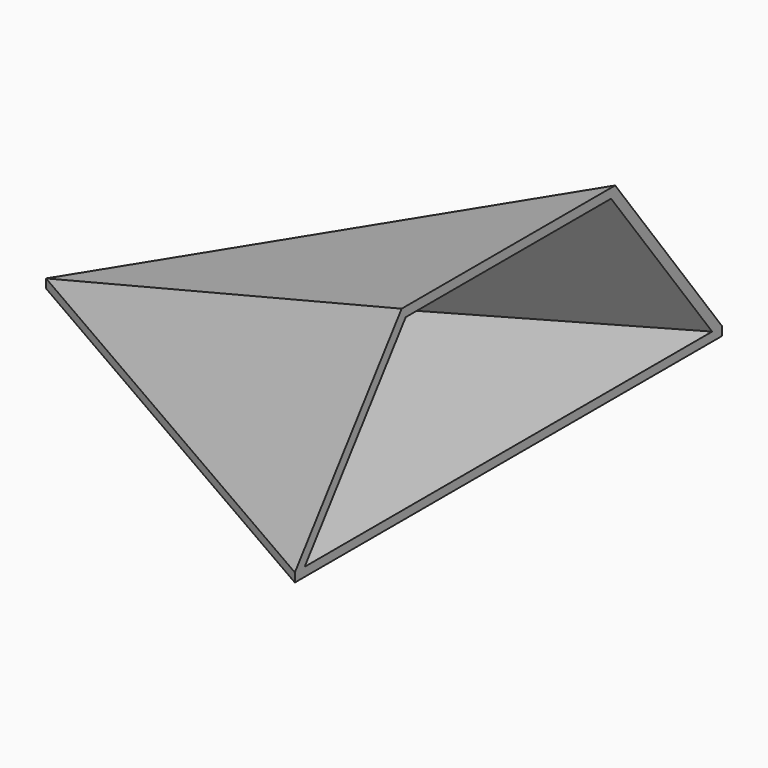
from build123d import *

# Parameters (mm, degrees)
F1_DEPTH = 2
F4_T     = -2


with BuildPart() as f1:
    # F0 (on Top) → F1 (new body)
    with BuildSketch(Plane.XY):
        Polygon((34.6410161514, -60), (34.6410161514, 60), (-69.2820323028, 0), align=None)
    extrude(amount=F1_DEPTH)

    # F2 (on face) → F3 section 0
    with BuildSketch(Plane.YZ.offset(34.6410161514), mode=Mode.PRIVATE) as f3_s0:
        Polygon((60, 2), (30, 42), (0, 42), (-30, 42), (-60, 2), align=None)
    loft([f3_s0.sketch, Vertex(-69.2820323028, 0, 2)])

    # F4
    f4_openings = [f1.faces().sort_by_distance(p)[0] for p in [
        (34.641016, 0, 18.604167),
    ]]
    offset(amount=F4_T, openings=f4_openings)


solid = f1.part
